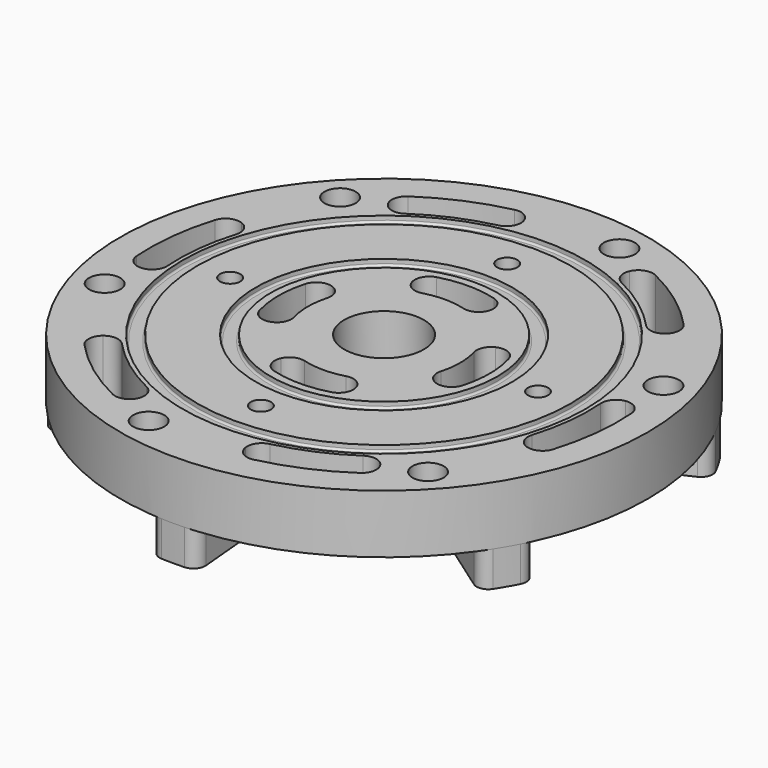
from build123d import *

# Parameters (mm, degrees)
F0_R             = 57.15
F1_DEPTH         = 12.7
F2_R             = 8.636
F3_DEPTH         = 12.701
F5_DEPTH         = 7.62
F6_T1_DEPTH      = 14.2671475518
F6_T3_DEPTH      = 13.7344913133
F8_COUNT         = 6
F9_D             = 4.3942
F9_DEPTH         = 15.24
F9_TIP           = 1.3201508661
F10_R            = 43.6245
F10_R_2          = 40.4241
F11_DEPTH        = 1.2954
F12_R            = 0.4064
F14_DEPTH        = 20.321
F14_COPIES_COUNT = 6
F15_R            = 3.17499
F16_R            = 27.7495
F16_R_2          = 24.5491
F17_DEPTH        = 1.2954
F18_R            = 0.4064
F20_DEPTH        = 20.321
F20_COPIES_COUNT = 4
F21_R            = 3.17499
F23_D            = 4.3942
F23_DEPTH        = 6.35
F23_TIP          = 1.3201508661
F25_D            = 6.7564


# Not quite as in the source:
# - a fillet or chamfer that OpenCascade refuses, or shapes differently, is made with other operations: its cross-section is extruded or revolved along the edge and cut away or added
# - a fillet or chamfer is up to 0.001 mm smaller than in the source, because OpenCascade refuses the exact size
# - a pattern or mirror of a feature is missing from the dataset's text; its kind, count and spacing are read off the source's solid


with BuildPart() as f1:
    # F0 (on Top) → F1 (new body)
    with BuildSketch(Plane.XY):
        Circle(F0_R)
    extrude(amount=F1_DEPTH)

    # F2 (on face) → F3 (cut, through all)
    with BuildSketch(Plane.XY.offset(12.7)):
        Circle(F2_R)
    extrude(amount=-F3_DEPTH, mode=Mode.SUBTRACT)

    # F4 (on face) → F5 (join)
    with BuildSketch(Plane(origin=(0, 0, 0), x_dir=(1, 0, 0), z_dir=(0, 0, -1))):
        with BuildLine():
            Line((-2.8575, -31.6211510504), (-5.1435, -56.9180718907))
            ThreePointArc((-5.1435, -56.9180718907), (0, -57.15), (5.1435, -56.9180718907))
            Line((5.1435, -56.9180718907), (2.8575, -31.6211510504))
            ThreePointArc((2.8575, -31.6211510504), (0, -31.75), (-2.8575, -31.6211510504))
        make_face()
    extrude(amount=F5_DEPTH)

    # F6: fillet of radius 2.54 on 4 edges, made by hand

    # F6_s2 → F6_t1 (cut)
    with BuildSketch(Plane.XY.offset(-14.2671475518)):
        with BuildLine():
            ThreePointArc((2.490581259, 57.0957047858), (4.2919178251, 56.2301660065), (4.9095808426, 54.3295179065))
            Line((4.9095808426, 54.3295179065), (5.1435, 56.9180718907))
            ThreePointArc((5.1435, 56.9180718907), (3.8180737982, 57.022318547), (2.490581259, 57.0957047858))
        make_face()
        with BuildLine():
            ThreePointArc((-2.490581259, 57.0957047858), (-4.2919178251, 56.2301660065), (-4.9095808426, 54.3295179065))
            Line((-4.9095808426, 54.3295179065), (-5.1435, 56.9180718907))
            ThreePointArc((-5.1435, 56.9180718907), (-3.8180737982, 57.022318547), (-2.490581259, 57.0957047858))
        make_face()
    extrude(amount=F6_T1_DEPTH, mode=Mode.SUBTRACT)

    # F6_s4 → F6_t3 (cut)
    with BuildSketch(Plane.XY.offset(-13.7344913133)):
        with BuildLine():
            ThreePointArc((0.5073422252, 31.7459462588), (2.2462164703, 32.396860006), (3.0776216873, 34.0570219595))
            Line((3.0776216873, 34.0570219595), (2.8575, 31.6211510504))
            ThreePointArc((2.8575, 31.6211510504), (1.6835778156, 31.7053318188), (0.5073422252, 31.7459462588))
        make_face()
        with BuildLine():
            ThreePointArc((-3.0776216873, 34.0570219595), (-2.2462164703, 32.396860006), (-0.5073422252, 31.7459462588))
            ThreePointArc((-0.5073422252, 31.7459462588), (-1.6835778156, 31.7053318188), (-2.8575, 31.6211510504))
            Line((-2.8575, 31.6211510504), (-3.0776216873, 34.0570219595))
        make_face()
    extrude(amount=F6_T3_DEPTH, mode=Mode.SUBTRACT)

    # F8: F1 ×6 about axis
    f8_axis = Axis((0, 0, 12.7), (0, 0, 1))


with BuildPart() as f1_1:
    add(f1.part)
    for i in range(1, F8_COUNT):
        add(f1.part.rotate(f8_axis, i * 360 / F8_COUNT))

    # F9
    with Locations(Plane(origin=(0, 0, -7.62), x_dir=(1, 0, 0), z_dir=(0, 0, -1))):
        with Locations((0, -50.8), (43.9940905122, -25.4), (43.9940905122, 25.4), (0, 50.8), (-43.9940905122, 25.4), (-43.9940905122, -25.4)):
            Hole(F9_D / 2, depth=F9_DEPTH)
            with Locations((0, 0, -(F9_DEPTH + F9_TIP / 2))):  # 118° drill point
                Cone(0, F9_D / 2, F9_TIP, mode=Mode.SUBTRACT)

    # F10 (on face) → F11 (cut)
    with BuildSketch(Plane.XY.offset(12.7)):
        Circle(F10_R)
        Circle(F10_R_2, mode=Mode.SUBTRACT)
    extrude(amount=-F11_DEPTH, mode=Mode.SUBTRACT)

    # F12
    f12_edges = [f1_1.edges().sort_by_distance(p)[0] for p in [
        (-43.6245, 0, 11.4046),
        (-40.4241, 0, 11.4046),
    ]]
    fillet(f12_edges, radius=F12_R)

    # F13 (on face) → F14 (cut, through all)
    with BuildSketch(Plane.XY.offset(12.7)):
        with BuildLine():
            ThreePointArc((16.721010174, 41.1850739803), (26.4387827868, 35.7322440487), (34.49502146, 28.0338365993))
            Line((34.49502146, 28.0338365993), (39.4228816685, 32.0386703992))
            ThreePointArc((39.4228816685, 32.0386703992), (30.2157517563, 40.8368503413), (19.1097259131, 47.0686559775))
            Line((19.1097259131, 47.0686559775), (16.721010174, 41.1850739803))
        make_face()
    f14 = extrude(amount=-F14_DEPTH, mode=Mode.SUBTRACT)

    # F14_copies: F14 ×6 about axis
    f14_copies_axis = Axis((0, 0, 0), (0, 0, 1))
    for i in range(1, F14_COPIES_COUNT):
        add(f14.rotate(f14_copies_axis, i * 360 / F14_COPIES_COUNT), mode=Mode.SUBTRACT)

    # F15 (radius 3.175 in the source; OpenCascade refuses exactly that, so slightly less here)
    f15_edges = [f1_1.edges().sort_by_distance(p)[0] for p in [
        (39.422882, 32.03867, 6.35),
        (19.109726, 47.068656, 6.35),
        (16.72101, 41.185074, 6.35),
        (34.495021, 28.033837, 6.35),
    ]]
    fillet(f15_edges, radius=F15_R)

    # F16 (on face) → F17 (cut)
    with BuildSketch(Plane.XY.offset(12.7)):
        Circle(F16_R)
        Circle(F16_R_2, mode=Mode.SUBTRACT)
    extrude(amount=-F17_DEPTH, mode=Mode.SUBTRACT)

    # F18
    f18_edges = [f1_1.edges().sort_by_distance(p)[0] for p in [
        (-27.7495, 0, 11.4046),
        (-24.5491, 0, 11.4046),
    ]]
    fillet(f18_edges, radius=F18_R)

    # F19 (on face) → F20 (cut, through all)
    with BuildSketch(Plane.XY.offset(12.7)):
        with BuildLine():
            Line((9.6610534634, -20.7181960117), (6.9774275013, -14.963141564))
            ThreePointArc((6.9774275013, -14.963141564), (0, -16.51), (-6.9774275013, -14.963141564))
            Line((-6.9774275013, -14.963141564), (-9.6610534634, -20.7181960117))
            ThreePointArc((-9.6610534634, -20.7181960117), (0, -22.86), (9.6610534634, -20.7181960117))
        make_face()
    f20 = extrude(amount=-F20_DEPTH, mode=Mode.SUBTRACT)

    # F20_copies: F20 ×4 about axis
    f20_copies_axis = Axis((0, 0, 0), (0, 0, 1))
    for i in range(1, F20_COPIES_COUNT):
        add(f20.rotate(f20_copies_axis, i * 360 / F20_COPIES_COUNT), mode=Mode.SUBTRACT)

    # F21 (radius 3.175 in the source; OpenCascade refuses exactly that, so slightly less here)
    f21_edges = [f1_1.edges().sort_by_distance(p)[0] for p in [
        (-6.977428, -14.963142, 6.35),
        (-9.661053, -20.718196, 6.35),
        (9.661053, -20.718196, 6.35),
        (6.977428, -14.963142, 6.35),
        (-20.718196, -9.661053, 6.35),
        (-20.718196, 9.661053, 6.35),
        (-14.963142, -6.977428, 6.35),
        (-14.963142, 6.977428, 6.35),
        (20.718196, 9.661053, 6.35),
        (20.718196, -9.661053, 6.35),
        (14.963142, -6.977428, 6.35),
        (14.963142, 6.977428, 6.35),
        (-9.661053, 20.718196, 6.35),
        (9.661053, 20.718196, 6.35),
        (6.977428, 14.963142, 6.35),
        (-6.977428, 14.963142, 6.35),
        (-16.72101, -41.185074, 6.35),
        (-19.109726, -47.068656, 6.35),
        (-39.422882, -32.03867, 6.35),
        (-34.495021, -28.033837, 6.35),
        (27.306815, -35.073357, 6.35),
        (31.207789, -40.083836, 6.35),
        (8.034862, -50.160552, 6.35),
        (7.030504, -43.890483, 6.35),
        (44.027825, 6.111717, 6.35),
        (50.317515, 6.98482, 6.35),
        (47.457743, -18.121882, 6.35),
        (41.525525, -15.856647, 6.35),
        (-44.027825, -6.111717, 6.35),
        (-50.317515, -6.98482, 6.35),
        (-47.457743, 18.121882, 6.35),
        (-41.525525, 15.856647, 6.35),
        (-27.306815, 35.073357, 6.35),
        (-31.207789, 40.083836, 6.35),
        (-8.034862, 50.160552, 6.35),
        (-7.030504, 43.890483, 6.35),
    ]]
    fillet(f21_edges, radius=F21_R)

    # F23
    with Locations(Plane.XY.offset(12.7)):
        with Locations((-33.3375, 0), (0, -33.3375), (33.3375, 0), (0, 33.3375)):
            Hole(F23_D / 2, depth=F23_DEPTH)
            with Locations((0, 0, -(F23_DEPTH + F23_TIP / 2))):  # 118° drill point
                Cone(0, F23_D / 2, F23_TIP, mode=Mode.SUBTRACT)

    # F25 (through all)
    with Locations(Plane.XY.offset(12.7)):
        with Locations((11.3576544358, 49.5140756323), (48.5592745603, 14.9210205473), (37.2016201245, -34.593055085), (-11.3576544358, -49.5140756323), (-48.5592745603, -14.9210205473), (-37.2016201245, 34.593055085)):
            Hole(F25_D / 2)


solid = f1_1.part
